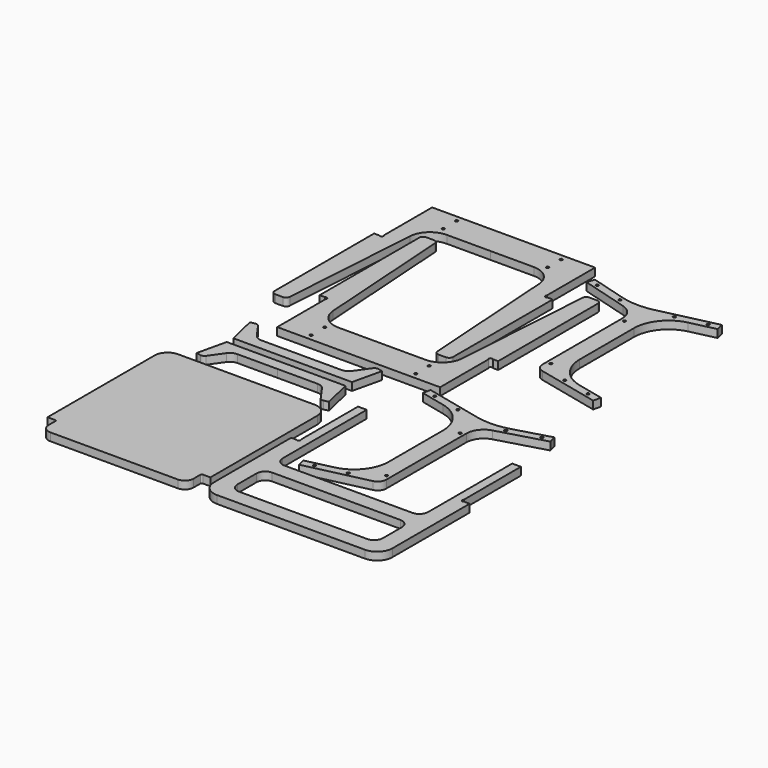
from build123d import *

# Parameters (mm, degrees)
F0_R     = 3
F1_DEPTH = 18


# Not quite as in the source:
# - ends of sketch curves that miss each other by under 0.0002 mm in the source are joined


with BuildPart() as f1:
    # F0 (on Top) → F1 (new body)
    with BuildSketch(Plane.XY):
        with BuildLine():
            Line((-2548.398753, 1864.9370212), (-2548.398753, 1578.9431252))
            ThreePointArc((-2548.398753, 1578.9431252), (-2545.7627143842, 1572.5791645229), (-2539.398754, 1569.9431252))
            Line((-2539.398754, 1569.9431252), (-2521.818432, 1569.9431252))
            ThreePointArc((-2521.818432, 1569.9431252), (-2515.6698935085, 1572.3707978561), (-2512.8383862489, 1578.3441291499))
            Line((-2512.8383862489, 1578.3441291499), (-2491.586816, 1896.9442072))
            ThreePointArc((-2491.586816, 1896.9442072), (-2476.3705560561, 1929.0443481057), (-2443.328871, 1942.0904452))
            Line((-2443.328871, 1942.0904452), (-2343.398753, 1942.0904332))
            Line((-2343.398753, 1942.0904332), (-2243.468642, 1942.0904452))
            ThreePointArc((-2243.468642, 1942.0904452), (-2210.4269542519, 1929.0443512004), (-2195.2106916665, 1896.9442102222))
            Line((-2195.2106916665, 1896.9442102222), (-2173.959121, 1578.3441292))
            ThreePointArc((-2173.959121, 1578.3441292), (-2171.1276142461, 1572.370798562), (-2164.979077, 1569.9431252))
            Line((-2164.979077, 1569.9431252), (-2147.398815, 1569.9431252))
            ThreePointArc((-2147.398815, 1569.9431252), (-2141.0348533229, 1572.5791638158), (-2138.398814, 1578.9431252))
            Line((-2138.398814, 1578.9431252), (-2138.398814, 1864.9370212))
            Line((-2138.398814, 1864.9370212), (-2150.74196, 1864.9370212))
            ThreePointArc((-2150.74196, 1864.9370212), (-2156.3988141247, 1864.9370210753), (-2156.3988141247, 1870.5938753247))
            Line((-2156.3988141247, 1870.5938753247), (-2156.398814, 2009.0000122))
            Line((-2156.398814, 2009.0000122), (-2530.398753, 2009.0000122))
            Line((-2530.398753, 2009.0000122), (-2530.398753, 1870.5938752))
            ThreePointArc((-2530.398753, 1870.5938752), (-2530.3987531252, 1864.9370208253), (-2536.0556076247, 1864.9370215753))
            Line((-2536.0556076247, 1864.9370215753), (-2548.398753, 1864.9370212))
        make_face()
        with Locations((-2463.398753, 1956.6404822)):
            Circle(F0_R, mode=Mode.SUBTRACT)
        with Locations((-2463.398753, 1995.5156652)):
            Circle(F0_R, mode=Mode.SUBTRACT)
        with Locations((-2223.398753, 1956.6404822)):
            Circle(F0_R, mode=Mode.SUBTRACT)
        with Locations((-2223.398753, 1995.5156652)):
            Circle(F0_R, mode=Mode.SUBTRACT)
    extrude(amount=F1_DEPTH)


with BuildPart() as f1b:
    # F0 (on Top) → F1, piece 2 (new body)
    with BuildSketch(Plane.XY):
        with BuildLine():
            ThreePointArc((-1995.045172, 1656.0524192), (-1990.6973347581, 1643.6021259909), (-1979.5441919006, 1636.5650176304))
            Line((-1979.5441919006, 1636.5650176304), (-1836.4784, 1603.5356652))
            Line((-1836.4784, 1603.5356652), (-1832.429266, 1621.0743312))
            Line((-1832.429266, 1621.0743312), (-1893.041255, 1635.0677182))
            ThreePointArc((-1893.041255, 1635.0677182), (-1937.6538240823, 1663.2161526833), (-1955.045172, 1713.0173242))
            Line((-1955.045172, 1713.0173242), (-1955.045172, 1868.4970762))
            ThreePointArc((-1955.045172, 1868.4970762), (-1937.6538241523, 1918.2982476287), (-1893.0412551083, 1946.4466816689))
            Line((-1893.0412551083, 1946.4466816689), (-1835.637701, 1959.6993462))
            Line((-1835.637701, 1959.6993462), (-1839.686774, 1977.2380122))
            Line((-1839.686774, 1977.2380122), (-1970.73349, 1946.9834862))
            ThreePointArc((-1970.73349, 1946.9834862), (-2008.4026894007, 1943.1903996148), (-2045.8217490169, 1948.949745141))
            Line((-2045.8217490169, 1948.949745141), (-2127.598028, 1972.3987182))
            Line((-2127.598028, 1972.3987182), (-2132.559454, 1955.0960142))
            Line((-2132.559454, 1955.0960142), (-2024.019677, 1923.9727202))
            ThreePointArc((-2024.019677, 1923.9727202), (-2003.0997501031, 1909.5948521421), (-1995.045172, 1885.5222492))
            Line((-1995.045172, 1885.5222492), (-1995.045172, 1656.0524192))
        make_face()
        with Locations((-1925.725775, 1633.3767602)):
            Circle(F0_R, mode=Mode.SUBTRACT)
        with Locations((-1985.545172, 1668.5608732)):
            Circle(F0_R, mode=Mode.SUBTRACT)
        with Locations((-1860.162115, 1618.2402252)):
            Circle(F0_R, mode=Mode.SUBTRACT)
        with Locations((-1985.545172, 1879.7423302)):
            Circle(F0_R, mode=Mode.SUBTRACT)
        with Locations((-2043.042486, 1938.7901212)):
            Circle(F0_R, mode=Mode.SUBTRACT)
        with Locations((-1925.725775, 1948.1376092)):
            Circle(F0_R, mode=Mode.SUBTRACT)
        with Locations((-2110.39234, 1958.1023772)):
            Circle(F0_R, mode=Mode.SUBTRACT)
        with Locations((-1860.162115, 1963.2741602)):
            Circle(F0_R, mode=Mode.SUBTRACT)
    extrude(amount=F1_DEPTH)


with BuildPart() as f1c:
    # F0 (on Top) → F1, piece 3 (new body)
    with BuildSketch(Plane.XY):
        with BuildLine():
            Line((-2065.094947, 1616.7593272), (-2065.094947, 1902.7532222))
            ThreePointArc((-2065.094947, 1902.7532222), (-2067.7309856158, 1909.1171838771), (-2074.094947, 1911.7532232))
            Line((-2074.094947, 1911.7532232), (-2091.675269, 1911.7532232))
            ThreePointArc((-2091.675269, 1911.7532232), (-2097.8238068809, 1909.3255501796), (-2100.6553137555, 1903.3522191837))
            Line((-2100.6553137555, 1903.3522191837), (-2121.906885, 1584.7521402))
            ThreePointArc((-2121.906885, 1584.7521402), (-2137.1231443325, 1552.6519999308), (-2170.164829, 1539.6059032))
            Line((-2170.164829, 1539.6059032), (-2270.094947, 1539.6059152))
            Line((-2270.094947, 1539.6059152), (-2370.025058, 1539.6059032))
            ThreePointArc((-2370.025058, 1539.6059032), (-2403.066745748, 1552.6519971996), (-2418.2830083334, 1584.7521381778))
            Line((-2418.2830083334, 1584.7521381778), (-2439.534579, 1903.3522192))
            ThreePointArc((-2439.534579, 1903.3522192), (-2442.3660861191, 1909.3255501796), (-2448.514624, 1911.7532232))
            Line((-2448.514624, 1911.7532232), (-2466.094886, 1911.7532232))
            ThreePointArc((-2466.094886, 1911.7532232), (-2472.4588470307, 1909.1171842307), (-2475.094886, 1902.7532232))
            Line((-2475.094886, 1902.7532232), (-2475.094886, 1616.7593272))
            Line((-2475.094886, 1616.7593272), (-2462.75174, 1616.7593272))
            ThreePointArc((-2462.75174, 1616.7593272), (-2457.0948858752, 1616.7593273247), (-2457.0948858752, 1611.1024730753))
            Line((-2457.0948858752, 1611.1024730753), (-2457.094886, 1472.6059152))
            Line((-2457.094886, 1472.6059152), (-2083.094947, 1472.6059152))
            Line((-2083.094947, 1472.6059152), (-2083.094947, 1611.1024732))
            ThreePointArc((-2083.094947, 1611.1024732), (-2083.0949471247, 1616.7593273247), (-2077.4380928752, 1616.7593273247))
            Line((-2077.4380928752, 1616.7593273247), (-2065.094947, 1616.7593272))
        make_face()
        with Locations((-2390.094947, 1486.1806832)):
            Circle(F0_R, mode=Mode.SUBTRACT)
        with Locations((-2390.094947, 1525.0558662)):
            Circle(F0_R, mode=Mode.SUBTRACT)
        with Locations((-2150.094947, 1486.1806832)):
            Circle(F0_R, mode=Mode.SUBTRACT)
        with Locations((-2150.094947, 1525.0558662)):
            Circle(F0_R, mode=Mode.SUBTRACT)
    extrude(amount=F1_DEPTH)


with BuildPart() as f1d:
    # F0 (on Top) → F1, piece 4 (new body)
    with BuildSketch(Plane.XY):
        with BuildLine():
            Line((-2092.743553, 1079.8126702), (-1949.67776, 1112.8419932))
            ThreePointArc((-1949.67776, 1112.8419932), (-1938.5246177944, 1119.8791002963), (-1934.17678, 1132.3293922))
            Line((-1934.17678, 1132.3293922), (-1934.17678, 1361.7992582))
            ThreePointArc((-1934.17678, 1361.7992582), (-1926.1222008996, 1385.8718584656), (-1905.2022758227, 1400.2497255816))
            Line((-1905.2022758227, 1400.2497255816), (-1796.662437, 1431.3730192))
            Line((-1796.662437, 1431.3730192), (-1801.623924, 1448.6757232))
            Line((-1801.623924, 1448.6757232), (-1883.400206, 1425.2267492))
            ThreePointArc((-1883.400206, 1425.2267492), (-1920.8192668385, 1419.4674045038), (-1958.488467047, 1423.2604929963))
            Line((-1958.488467047, 1423.2604929963), (-2089.535179, 1453.5150172))
            Line((-2089.535179, 1453.5150172), (-2093.584312, 1435.9763512))
            Line((-2093.584312, 1435.9763512), (-2036.1807, 1422.7236872))
            ThreePointArc((-2036.1807, 1422.7236872), (-1991.5681310063, 1394.5752565997), (-1974.17678, 1344.7740882))
            Line((-1974.17678, 1344.7740882), (-1974.17678, 1189.2943072))
            ThreePointArc((-1974.17678, 1189.2943072), (-1991.5681310063, 1139.4931388003), (-2036.1806999591, 1111.3447080229))
            Line((-2036.1806999591, 1111.3447080229), (-2096.792686, 1097.3513052))
            Line((-2096.792686, 1097.3513052), (-2092.743553, 1079.8126702))
        make_face()
        with Locations((-2069.059837, 1094.5172302)):
            Circle(F0_R, mode=Mode.SUBTRACT)
        with Locations((-2003.496177, 1109.6537962)):
            Circle(F0_R, mode=Mode.SUBTRACT)
        with Locations((-1943.67678, 1144.8378782)):
            Circle(F0_R, mode=Mode.SUBTRACT)
        with Locations((-1943.67678, 1356.0193432)):
            Circle(F0_R, mode=Mode.SUBTRACT)
        with Locations((-1886.179466, 1415.0671262)):
            Circle(F0_R, mode=Mode.SUBTRACT)
        with Locations((-2003.496177, 1424.4146142)):
            Circle(F0_R, mode=Mode.SUBTRACT)
        with Locations((-2069.059837, 1439.5511652)):
            Circle(F0_R, mode=Mode.SUBTRACT)
        with Locations((-1818.829612, 1434.3793822)):
            Circle(F0_R, mode=Mode.SUBTRACT)
    extrude(amount=F1_DEPTH)


with BuildPart() as f1e:
    # F0 (on Top) → F1, piece 5 (new body)
    with BuildSketch(Plane.XY):
        with BuildLine():
            Line((-2496.867429, 1458.8053732), (-2506.994856, 1456.4671952))
            Line((-2506.994856, 1456.4671952), (-2491.55229, 1389.5781572))
            Line((-2491.55229, 1389.5781572), (-2218.960997, 1389.5781572))
            Line((-2218.960997, 1389.5781572), (-2203.518431, 1456.4671952))
            Line((-2203.518431, 1456.4671952), (-2213.645843, 1458.8053732))
            ThreePointArc((-2213.645843, 1458.8053732), (-2219.1088864644, 1458.4300973777), (-2223.4363526287, 1455.0746969373))
            Line((-2223.4363526287, 1455.0746969373), (-2245.428739, 1423.9921952))
            ThreePointArc((-2245.428739, 1423.9921952), (-2253.3795764291, 1417.0711218333), (-2263.621763, 1414.5781942))
            Line((-2263.621763, 1414.5781942), (-2355.256636, 1414.5781572))
            Line((-2355.256636, 1414.5781572), (-2446.891501, 1414.5781942))
            ThreePointArc((-2446.891501, 1414.5781942), (-2457.1336878274, 1417.0711219661), (-2465.0845255903, 1423.9921954899))
            Line((-2465.0845255903, 1423.9921954899), (-2487.076919, 1455.0746972))
            ThreePointArc((-2487.076919, 1455.0746972), (-2491.4043855356, 1458.4300973777), (-2496.867429, 1458.8053732))
        make_face()
    extrude(amount=F1_DEPTH)


with BuildPart() as f1f:
    # F0 (on Top) → F1, piece 6 (new body)
    with BuildSketch(Plane.XY):
        with BuildLine():
            ThreePointArc((-2529.999997, 1279.2192542), (-2551.2132020214, 1270.4324590498), (-2560, 1249.2192552))
            Line((-2560, 1249.2192552), (-2560, 942.0285802))
            Line((-2560, 942.0285802), (-2542.5, 942.0285802))
            ThreePointArc((-2542.5, 942.0285802), (-2540.3786796564, 941.1499005436), (-2539.5, 939.0285802))
            Line((-2539.5, 939.0285802), (-2539.5, 919.2192552))
            ThreePointArc((-2539.5, 919.2192552), (-2533.6421359773, 905.0771189298), (-2519.5, 899.2192542))
            Line((-2519.5, 899.2192542), (-2226.5, 899.2192542))
            ThreePointArc((-2226.5, 899.2192542), (-2212.3578640227, 905.0771189298), (-2206.5, 919.2192552))
            Line((-2206.5, 919.2192552), (-2206.5, 939.0285802))
            ThreePointArc((-2206.5, 939.0285802), (-2205.6213203436, 941.1499005436), (-2203.5, 942.0285802))
            Line((-2203.5, 942.0285802), (-2186, 942.0285802))
            Line((-2186, 942.0285802), (-2186, 1249.2192552))
            ThreePointArc((-2186, 1249.2192552), (-2194.7867979786, 1270.4324590498), (-2216.000003, 1279.2192542))
            Line((-2216.000003, 1279.2192542), (-2529.999997, 1279.2192542))
        make_face()
    extrude(amount=F1_DEPTH)


with BuildPart() as f1g:
    # F0 (on Top) → F1, piece 7 (new body)
    with BuildSketch(Plane.XY):
        with BuildLine():
            Line((-2131.118722, 1322.0958222), (-2151.118722, 1322.0958222))
            Line((-2151.118722, 1322.0958222), (-2151.118722, 1158.1837612))
            ThreePointArc((-2151.118722, 1158.1837612), (-2151.1187216252, 1152.5269063253), (-2156.7755761247, 1152.5269060753))
            Line((-2156.7755761247, 1152.5269060753), (-2169.118722, 1152.5269062))
            Line((-2169.118722, 1152.5269062), (-2169.118722, 930.8199362))
            ThreePointArc((-2169.118722, 930.8199362), (-2158.8674600486, 906.0711995656), (-2134.118724, 895.8199362))
            Line((-2134.118724, 895.8199362), (-1794.118724, 895.8199362))
            ThreePointArc((-1794.118724, 895.8199362), (-1769.3699853656, 906.0711981514), (-1759.118722, 930.8199362))
            Line((-1759.118722, 930.8199362), (-1759.118722, 1152.5269062))
            Line((-1759.118722, 1152.5269062), (-1771.461867, 1152.5269062))
            ThreePointArc((-1771.461867, 1152.5269062), (-1777.1187221247, 1152.5269060753), (-1777.1187216247, 1158.1837608247))
            Line((-1777.1187216247, 1158.1837608247), (-1777.118722, 1322.0958222))
            Line((-1777.118722, 1322.0958222), (-1797.118722, 1322.0958222))
            Line((-1797.118722, 1322.0958222), (-1797.118722, 1080.8199362))
            ThreePointArc((-1797.118722, 1080.8199362), (-1802.9765867298, 1066.6778002227), (-1817.118723, 1060.8199362))
            Line((-1817.118723, 1060.8199362), (-2111.118723, 1060.8199362))
            ThreePointArc((-2111.118723, 1060.8199362), (-2125.2608576237, 1066.6778005763), (-2131.118722, 1080.8199352))
            Line((-2131.118722, 1080.8199352), (-2131.118722, 1322.0958222))
        make_face()
        with BuildLine():
            Line((-2131.118722, 950.8199382), (-2131.118722, 1005.8199382))
            ThreePointArc((-2131.118722, 1005.8199382), (-2125.2608572702, 1019.9620721773), (-2111.118723, 1025.8199362))
            Line((-2111.118723, 1025.8199362), (-1817.118723, 1025.8199362))
            ThreePointArc((-1817.118723, 1025.8199362), (-1802.9765867298, 1019.9620721773), (-1797.118722, 1005.8199362))
            Line((-1797.118722, 1005.8199362), (-1797.118722, 950.8199362))
            ThreePointArc((-1797.118722, 950.8199362), (-1802.9765867298, 936.6778002227), (-1817.118723, 930.8199362))
            Line((-1817.118723, 930.8199362), (-2111.118723, 930.8199362))
            ThreePointArc((-2111.118723, 930.8199362), (-2125.2608586844, 936.6778016369), (-2131.118722, 950.8199382))
        make_face(mode=Mode.SUBTRACT)
    extrude(amount=F1_DEPTH)


with BuildPart() as f1h:
    # F0 (on Top) → F1, piece 8 (new body)
    with BuildSketch(Plane.XY):
        with BuildLine():
            ThreePointArc((-2465.0845255903, 1336.4825670837), (-2457.1336878274, 1343.4036406075), (-2446.891501, 1345.8965683736))
            Line((-2446.891501, 1345.8965683736), (-2355.256636, 1345.8966053736))
            Line((-2355.256636, 1345.8966053736), (-2263.621763, 1345.8965683736))
            ThreePointArc((-2263.621763, 1345.8965683736), (-2253.3795764291, 1343.4036407403), (-2245.4287387433, 1336.4825675552))
            Line((-2245.4287387433, 1336.4825675552), (-2223.436353, 1305.4000653736))
            ThreePointArc((-2223.436353, 1305.4000653736), (-2219.1088864644, 1302.0446651959), (-2213.6458430225, 1301.6693894709))
            Line((-2213.6458430225, 1301.6693894709), (-2203.518431, 1304.0075673736))
            Line((-2203.518431, 1304.0075673736), (-2218.960997, 1370.8966053736))
            Line((-2218.960997, 1370.8966053736), (-2491.55229, 1370.8966053736))
            Line((-2491.55229, 1370.8966053736), (-2506.994856, 1304.0075673736))
            Line((-2506.994856, 1304.0075673736), (-2496.867429, 1301.6693893736))
            ThreePointArc((-2496.867429, 1301.6693893736), (-2491.4043855356, 1302.0446651959), (-2487.0769193713, 1305.4000656363))
            Line((-2487.0769193713, 1305.4000656363), (-2465.0845255903, 1336.4825670837))
        make_face()
    extrude(amount=F1_DEPTH)


solid = Compound([f1.part, f1b.part, f1c.part, f1d.part, f1e.part, f1f.part, f1g.part, f1h.part])
